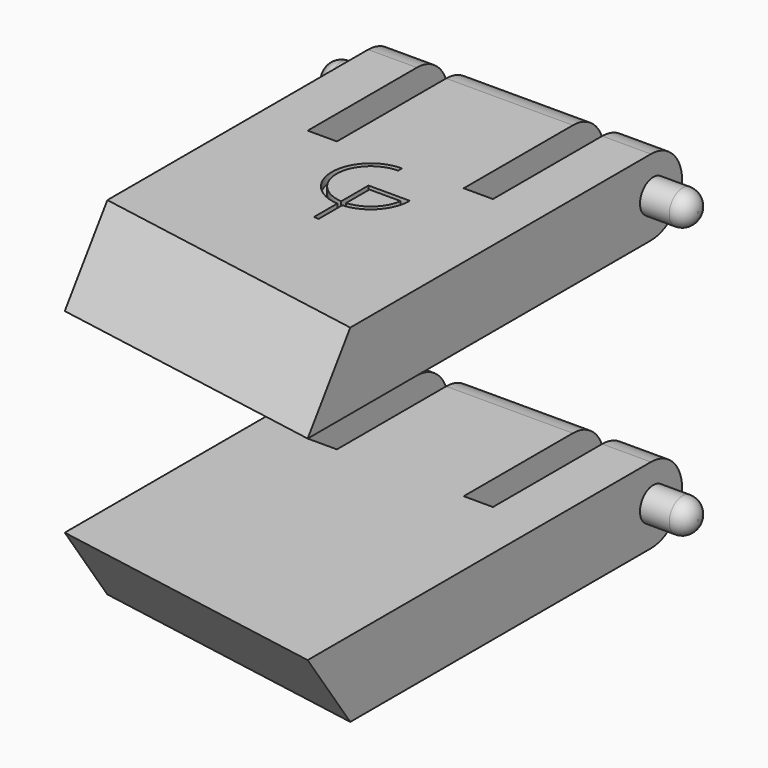
from build123d import *

# Parameters (mm, degrees)
F1_DEPTH    = 3.9
F2_R        = 0.85
F3_DEPTH    = 2.3
F4_R        = 0.85
F5_DEPTH    = 2.3
F6_R        = 0.8
F7_T1_DEPTH = 12.5
F7_T3_DEPTH = 12.5
F13_DEPTH   = 0.4
F15_DEPTH   = 0.4


# Not quite as in the source:
# - a fillet or chamfer that OpenCascade refuses, or shapes differently, is made with other operations: its cross-section is extruded or revolved along the edge and cut away or added
# - a feature names something its author has since deleted; it is built from what else it names


with BuildPart() as f1:
    # F0 (on Top) → F1 (new body)
    with BuildSketch(Plane.XY):
        Polygon((-14.5, 2.5567412203), (0, 0), (0, 24), (-2.5, 24), (-2.5, 15), (-4, 15), (-4, 24), (-10.5, 24), (-10.5, 15), (-12, 15), (-12, 24), (-14.5, 24), align=None)
    extrude(amount=F1_DEPTH)

    # F2 (on face) → F3 (join)
    with BuildSketch(Plane.YZ):
        with Locations((22.15, 1.95)):
            Circle(F2_R)
    extrude(amount=F3_DEPTH)

    # F4 (on face) → F5 (join)
    with BuildSketch(Plane(origin=(-14.5, 0, 0), x_dir=(0, -1, 0), z_dir=(-1, 0, 0))):
        with Locations((-22.15, 1.95)):
            Circle(F4_R)
    extrude(amount=F5_DEPTH)

    # F6
    f6_edges = [f1.edges().sort_by_distance(p)[0] for p in [
        (2.3, 21.3, 1.95),
        (-16.8, 23, 1.95),
    ]]
    fillet(f6_edges, radius=F6_R)

    # F7: fillet of radius 2 on 4 edges, made by hand

    # F7_s2 → F7_t1 (cut)
    with BuildSketch(Plane.YZ.offset(-19.5)):
        with BuildLine():
            ThreePointArc((24, 1.9), (23.4142135624, 3.3142135624), (22, 3.9))
            Line((22, 3.9), (24, 3.9))
            Line((24, 3.9), (24, 1.9))
        make_face()
        with BuildLine():
            ThreePointArc((24, 2), (23.4142135624, 0.5857864376), (22, 0))
            Line((22, 0), (24, 0))
            Line((24, 0), (24, 2))
        make_face()
    extrude(amount=F7_T1_DEPTH, mode=Mode.SUBTRACT)

    # F7_s4 → F7_t3 (cut)
    with BuildSketch(Plane.YZ.offset(-7.5)):
        with BuildLine():
            ThreePointArc((22, 3.9), (23.4142135624, 3.3142135624), (24, 1.9))
            Line((24, 1.9), (24, 3.9))
            Line((24, 3.9), (22, 3.9))
        make_face()
        with BuildLine():
            ThreePointArc((22, 0), (23.4142135624, 0.5857864376), (24, 2))
            Line((24, 2), (24, 0))
            Line((24, 0), (22, 0))
        make_face()
    extrude(amount=F7_T3_DEPTH, mode=Mode.SUBTRACT)

    # F9: sweep along a path in F9_path
    with BuildLine(Plane(origin=(0, 0, 3.9), x_dir=(0.984807753, -0.1736481777, 0), z_dir=(0.1736481777, 0.984807753, 0))) as f9_path:
        Line((0, 0), (-14.7236858723, 0))
    # F8 (on face) → F9 (sweep, cut)
    with BuildSketch(Plane.YZ):
        Polygon((0, 3.9), (0, 0), (2.730809399, 3.9), align=None)
    sweep(path=f9_path.line, mode=Mode.SUBTRACT)


with BuildPart() as f1_1:
    # F10: moved
    add(f1.part.moved(Location((0, 0, 5))))


with BuildPart() as f11_1:
    # F11: instance of F1
    add(f1_1.part.mirror(Plane.XY))

    # F14 (on face) → F15 (cut)
    with BuildSketch(Plane(origin=(0, 0, -8.9), x_dir=(1, 0, 0), z_dir=(0, 0, -1))):
        with BuildLine():
            Line((-7.0138571055, -14.382870473), (-7.0138571055, -14.632870473))
            ThreePointArc((-7.0138571055, -14.632870473), (-5.0147581199, -12.6928975156), (-6.8938571055, -10.6364737188))
            Line((-6.8938571055, -10.6364737188), (-6.8938571055, -10.8869896065))
            ThreePointArc((-6.8938571055, -10.8869896065), (-5.264887192, -12.692905811), (-7.0138571055, -14.382870473))
        make_face()
        with BuildLine():
            Line((-6.8938571055, -12.632870473), (-6.8938571055, -10.8869896065))
            ThreePointArc((-6.8938571055, -10.8869896065), (-7.0188699097, -10.8828776525), (-7.1438571055, -10.8877057243))
            Line((-7.1438571055, -10.8877057243), (-7.1438571055, -12.382870473))
            Line((-7.1438571055, -12.382870473), (-8.745907913, -12.382870473))
            ThreePointArc((-8.745907913, -12.382870473), (-8.7593640395, -12.5075487136), (-8.7638571055, -12.632870473))
            Line((-8.7638571055, -12.632870473), (-6.8938571055, -12.632870473))
        make_face()
        with BuildLine():
            Line((-7.1438571055, -10.8877057243), (-7.1438571055, -10.6370999451))
            ThreePointArc((-7.1438571055, -10.6370999451), (-8.4733090574, -11.2653910398), (-9.0138571055, -12.632870473))
            Line((-9.0138571055, -12.632870473), (-8.7638571055, -12.632870473))
            ThreePointArc((-8.7638571055, -12.632870473), (-8.7593640395, -12.5075487136), (-8.745907913, -12.382870473))
            ThreePointArc((-8.745907913, -12.382870473), (-8.2078787589, -11.3534908221), (-7.1438571055, -10.8877057243))
        make_face()
        with BuildLine():
            Line((-6.8938571055, -10.8869896065), (-6.8938571055, -10.6364737188))
            ThreePointArc((-6.8938571055, -10.6364737188), (-7.0188668999, -10.6328767475), (-7.1438571055, -10.6370999451))
            Line((-7.1438571055, -10.6370999451), (-7.1438571055, -10.8877057243))
            ThreePointArc((-7.1438571055, -10.8877057243), (-7.0188699097, -10.8828776525), (-6.8938571055, -10.8869896065))
        make_face()
        with BuildLine():
            ThreePointArc((-7.1438571055, -10.6370999451), (-7.0188668999, -10.6328767475), (-6.8938571055, -10.6364737188))
            Line((-6.8938571055, -10.6364737188), (-6.8938571055, -9.132870473))
            Line((-6.8938571055, -9.132870473), (-7.1438571055, -9.132870473))
            Line((-7.1438571055, -9.132870473), (-7.1438571055, -10.6370999451))
        make_face()
    extrude(amount=-F15_DEPTH, mode=Mode.SUBTRACT)


with BuildPart() as f1_2:
    add(f1_1.part)

    # F12 (on face) → F13 (cut)
    with BuildSketch(Plane.XY.offset(8.9)):
        with BuildLine():
            Line((-7.0054624054, 14.5548715198), (-7.0054624054, 14.8048715198))
            ThreePointArc((-7.0054624054, 14.8048715198), (-9.004561391, 12.8648985624), (-7.1254624054, 10.8084747656))
            Line((-7.1254624054, 10.8084747656), (-7.1254624054, 11.0589906533))
            ThreePointArc((-7.1254624054, 11.0589906533), (-8.7544323188, 12.8649068578), (-7.0054624054, 14.5548715198))
        make_face()
        with BuildLine():
            Line((-6.8754624054, 11.0597067711), (-6.8754624054, 10.8091009919))
            ThreePointArc((-6.8754624054, 10.8091009919), (-5.5460104535, 11.4373920867), (-5.0054624054, 12.8048715198))
            Line((-5.0054624054, 12.8048715198), (-5.2554624054, 12.8048715198))
            ThreePointArc((-5.2554624054, 12.8048715198), (-5.2599554714, 12.6795497604), (-5.2734115978, 12.5548715198))
            ThreePointArc((-5.2734115978, 12.5548715198), (-5.8114407519, 11.5254918689), (-6.8754624054, 11.0597067711))
        make_face()
        with BuildLine():
            Line((-7.1254624054, 12.8048715198), (-7.1254624054, 11.0589906533))
            ThreePointArc((-7.1254624054, 11.0589906533), (-7.0004496012, 11.0548786993), (-6.8754624054, 11.0597067711))
            Line((-6.8754624054, 11.0597067711), (-6.8754624054, 12.5548715198))
            Line((-6.8754624054, 12.5548715198), (-5.2734115978, 12.5548715198))
            ThreePointArc((-5.2734115978, 12.5548715198), (-5.2599554714, 12.6795497604), (-5.2554624054, 12.8048715198))
            Line((-5.2554624054, 12.8048715198), (-7.1254624054, 12.8048715198))
        make_face()
        with BuildLine():
            Line((-7.1254624054, 11.0589906533), (-7.1254624054, 10.8084747656))
            ThreePointArc((-7.1254624054, 10.8084747656), (-7.000452611, 10.8048777943), (-6.8754624054, 10.8091009919))
            Line((-6.8754624054, 10.8091009919), (-6.8754624054, 11.0597067711))
            ThreePointArc((-6.8754624054, 11.0597067711), (-7.0004496012, 11.0548786993), (-7.1254624054, 11.0589906533))
        make_face()
        with BuildLine():
            ThreePointArc((-6.8754624054, 10.8091009919), (-7.000452611, 10.8048777943), (-7.1254624054, 10.8084747656))
            Line((-7.1254624054, 10.8084747656), (-7.1254624054, 9.3048715198))
            Line((-7.1254624054, 9.3048715198), (-6.8754624054, 9.3048715198))
            Line((-6.8754624054, 9.3048715198), (-6.8754624054, 10.8091009919))
        make_face()
    extrude(amount=-F13_DEPTH, mode=Mode.SUBTRACT)


solid = Compound([f11_1.part, f1_2.part])
